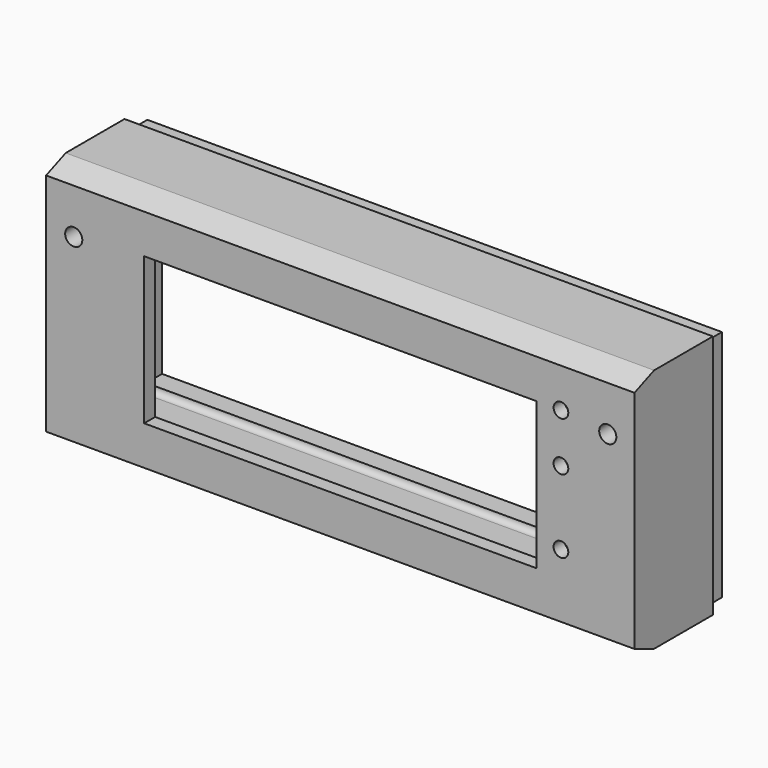
from build123d import *

# Parameters (mm, degrees)
F0_W          = 120
F0_H          = 50
F1_DEPTH      = 10
F1_DEPTH_BACK = 10
F2_T          = -2.8
F3_W          = 80
F3_H          = 30
F4_DEPTH      = 20.001
F6_W          = 5
F6_H          = 10
F7_DEPTH      = 7.2
F8_F1_R       = 2
F8_F2_R       = 2
F9_SIZE2      = 2
F9_SIZE       = 5
F9_2_SIZE2    = 2
F9_2_SIZE     = 5
F10_D         = 3
F12_D         = 3.5
F12_DEPTH     = 5
F12_START     = 5.9405501
F12_TIP       = 1.0515060833
F13_W         = 117.182782799
F13_H         = 47.6424540132
F13_W_2       = 111.182782799
F13_H_2       = 41.6424540132
F14_DEPTH     = 4
F15_R         = 1.2


with BuildPart() as f1:
    # F0 (on Front) → F1 (new body, two sides)
    with BuildSketch(Plane.XZ) as f1_sk:
        Rectangle(F0_W, F0_H)
    extrude(amount=F1_DEPTH)
    extrude(f1_sk.sketch, amount=-F1_DEPTH_BACK)

    # F2
    f2_openings = [f1.faces().sort_by_distance(p)[0] for p in [
        (0, 10, 0),
    ]]
    offset(amount=F2_T, openings=f2_openings)

    # F3 (on face) → F4 (cut, through all)
    with BuildSketch(Plane.XZ.offset(10)):
        Rectangle(F3_W, F3_H)
    extrude(amount=-F4_DEPTH, mode=Mode.SUBTRACT)

    # F6 (on Front) → F7 (join, through all)
    with BuildSketch(Plane.XZ):
        with Locations((54.7, 17.2)):
            Rectangle(F6_W, F6_H)
        with Locations((54.7, -17.2)):
            Rectangle(F6_W, F6_H)
        with Locations((-54.7, 17.2)):
            Rectangle(F6_W, F6_H)
        with Locations((-54.7, -17.2)):
            Rectangle(F6_W, F6_H)
    extrude(amount=F7_DEPTH)

    # F8: fillet of radius 2 on 14 edges, made by hand

    # F8_f1
    f8_f1_edges = [f1.edges().sort_by_distance(p)[0] for p in [
        (52.2, -3.6, 12.2),
        (-52.2, -3.6, 12.2),
        (-52.2, -3.6, -12.2),
        (52.2, -3.6, -12.2),
    ]]
    fillet(f8_f1_edges, radius=F8_F1_R)

    # F8_f2
    f8_f2_edges = [f1.edges().sort_by_distance(p)[0] for p in [
        (52.2, -7.2, -18.2),
        (52.2, -7.2, 18.2),
        (0, -7.2, 22.2),
        (-52.2, -7.2, 18.2),
        (-52.2, -3.6, 22.2),
        (-57.2, -3.6, 12.2),
        (-57.2, -7.2, 0),
        (0, -7.2, -22.2),
        (-52.2, -7.2, -18.2),
        (-52.2, -3.6, -22.2),
        (-52.7857864376, -7.2, -12.7857864376),
        (-52.7857864376, -7.2, 12.7857864376),
        (52.7857864376, -7.2, 12.7857864376),
        (52.7857864376, -7.2, -12.7857864376),
    ]]
    fillet(f8_f2_edges, radius=F8_F2_R)

    # F9
    f9_edges = [f1.edges().sort_by_distance(p)[0] for p in [
        (0, -10, -25),
    ]]
    f9_side = f1.faces().sort_by_distance((0, 0, -25))[0]
    chamfer(f9_edges, length=F9_SIZE, length2=F9_SIZE2, reference=f9_side)

    # F9#2
    f9_2_edges = [f1.edges().sort_by_distance(p)[0] for p in [
        (0, -10, 25),
    ]]
    f9_2_side = f1.faces().sort_by_distance((0, 0, 25))[0]
    chamfer(f9_2_edges, length=F9_2_SIZE, length2=F9_2_SIZE2, reference=f9_2_side)

    # F10 (through all)
    with Locations(Plane.XZ.offset(10)):
        with Locations((45, 5), (45, 15), (45, -10)):
            Hole(F10_D / 2)

    # F12
    # its depths count from where the whole tool has entered the part; down to there all is cleared
    with Locations(Plane(origin=(0, 0, 0), x_dir=(1, 0, 0), z_dir=(0, 1, 0))):
        with Locations((54.5504838228, -13.8078443706), (-54.356444627, -13.8078443706)):
            Hole(F12_D / 2, depth=F12_START)
    with Locations(Plane(origin=(0, 0, 0), x_dir=(1, 0, 0), z_dir=(0, 1, 0))):
        with Locations((54.5504838228, -13.8078443706, -F12_START), (-54.356444627, -13.8078443706, -F12_START), (-54.356444627, 15.7220419496, 0), (54.5504838228, 15.7220419496, 0)):
            Hole(F12_D / 2, depth=F12_DEPTH)
            with Locations((0, 0, -(F12_DEPTH + F12_TIP / 2))):  # 118° drill point
                Cone(0, F12_D / 2, F12_TIP, mode=Mode.SUBTRACT)

    # F13 (on face) → F14 (join)
    with BuildSketch(Plane(origin=(0, 10, 0), x_dir=(-1, 0, 0), z_dir=(0, 1, 0))):
        with Locations((-0.0398587435, -0.1178945079)):
            Rectangle(F13_W, F13_H)
        with Locations((-0.0398587435, -0.1178945079)):
            Rectangle(F13_W_2, F13_H_2, mode=Mode.SUBTRACT)
    extrude(amount=F14_DEPTH)

    # F15
    f15_edges = [f1.edges().sort_by_distance(p)[0] for p in [
        (0, 10, 22.2),
        (-57.2, 10, 0),
        (0, 10, -22.2),
        (57.2, 10, 0),
    ]]
    fillet(f15_edges, radius=F15_R)


solid = f1.part
